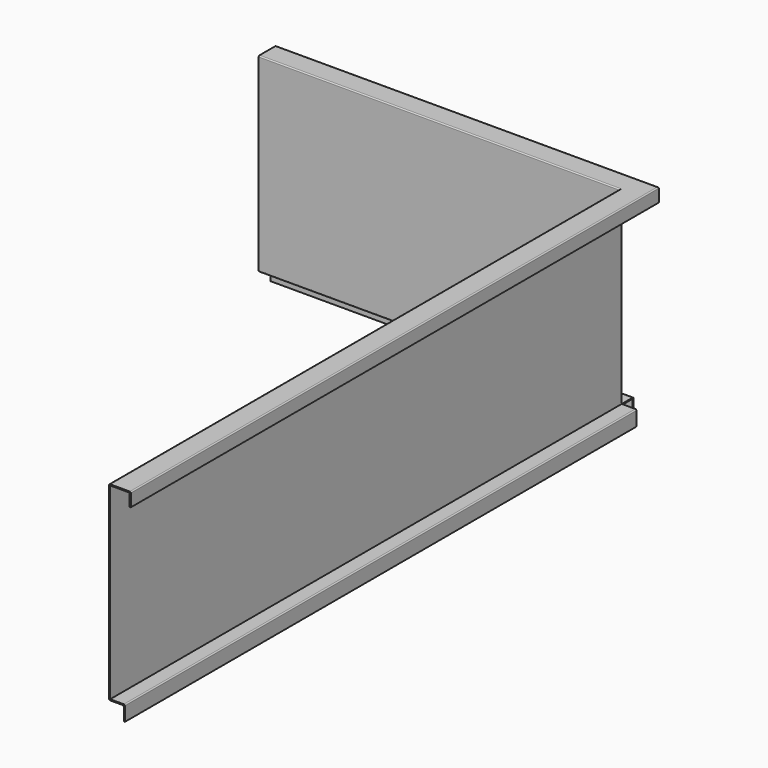
from build123d import *

# Parameters (mm, degrees)
F3_W         = 27
F3_H         = 27
F4_DEPTH     = 30
F5_T1_DEPTH  = 666
F5_T3_DEPTH  = 702
F5_T5_DEPTH  = 1176
F5_T7_DEPTH  = 1212
F5_T13_DEPTH = 1181
F5_T17_DEPTH = 671
F5_T20_DEPTH = 669
F5_T22_DEPTH = 676
F5_T24_DEPTH = 714
F5_T26_DEPTH = 1224
F5_T28_DEPTH = 1179
F5_T30_DEPTH = 1186
F5_T36_DEPTH = 674
F5_T40_DEPTH = 1184
F5_T47_DEPTH = 674
F5_T51_DEPTH = 1184


# Not quite as in the source:
# - a fillet or chamfer that OpenCascade refuses, or shapes differently, is made with other operations: its cross-section is extruded or revolved along the edge and cut away or added


with BuildPart() as f2:
    # F2: sweep along a path in F1
    with BuildLine(Plane.XY) as f2_path:
        Line((0, 0), (0, 1174))
        Line((0, 1174), (-664, 1174))
    # F0 (on Front) → F2 (sweep)
    with BuildSketch(Plane.XZ):
        Polygon((38, -2), (38, -25), (40, -25), (40, 0), (0, 0), (0, -350), (27, -350), (27, -376), (29, -376), (29, -348), (2, -348), (2, -2), align=None)
    sweep(path=f2_path.line, transition=Transition.RIGHT)

    # F3 (on face) → F4 (cut)
    with BuildSketch(Plane.XY.offset(-348)):
        with Locations((15.5, 1189.5)):
            Rectangle(F3_W, F3_H)
    extrude(amount=-F4_DEPTH, mode=Mode.SUBTRACT)

    # F5: fillet of radius 2 on 15 edges, made by hand

    # F5_s2 → F5_t1 (join)
    with BuildSketch(Plane.YZ.offset(-664)):
        with BuildLine():
            ThreePointArc((1199, -350), (1200.4142135624, -350.5857864376), (1201, -352))
            Line((1201, -352), (1201, -350))
            Line((1201, -350), (1199, -350))
        make_face()
        with BuildLine():
            ThreePointArc((1176, -346), (1176.5857864376, -347.4142135624), (1178, -348))
            Line((1178, -348), (1176, -348))
            Line((1176, -348), (1176, -346))
        make_face()
        with BuildLine():
            ThreePointArc((1178, -2), (1176.5857864376, -2.5857864376), (1176, -4))
            Line((1176, -4), (1176, -2))
            Line((1176, -2), (1178, -2))
        make_face()
    extrude(amount=F5_T1_DEPTH)

    # F5_s4 → F5_t3 (join)
    with BuildSketch(Plane.YZ.offset(-664)):
        with BuildLine():
            ThreePointArc((1210, -2), (1211.4142135624, -2.5857864376), (1212, -4))
            Line((1212, -4), (1212, -2))
            Line((1212, -2), (1210, -2))
        make_face()
    extrude(amount=F5_T3_DEPTH)

    # F5_s6 → F5_t5 (join)
    with BuildSketch(Plane.XZ.offset(-1176)):
        with BuildLine():
            ThreePointArc((25, -350), (26.4142135624, -350.5857864376), (27, -352))
            Line((27, -352), (27, -350))
            Line((27, -350), (25, -350))
        make_face()
        with BuildLine():
            ThreePointArc((4, -2), (2.5857864376, -2.5857864376), (2, -4))
            Line((2, -4), (2, -2))
            Line((2, -2), (4, -2))
        make_face()
    extrude(amount=F5_T5_DEPTH)

    # F5_s8 → F5_t7 (join)
    with BuildSketch(Plane.XZ.offset(-1212)):
        with BuildLine():
            ThreePointArc((38, -4), (37.4142135624, -2.5857864376), (36, -2))
            Line((36, -2), (38, -2))
            Line((38, -2), (38, -4))
        make_face()
    extrude(amount=F5_T7_DEPTH)


with BuildPart() as f5_tool11:
    # F5_s12 → F5_t13 (new body)
    with BuildSketch(Plane.XZ):
        with BuildLine():
            ThreePointArc((4, -2), (2.5857864376, -2.5857864376), (2, -4))
            Line((2, -4), (2, -2))
            Line((2, -2), (4, -2))
        make_face()
    extrude(amount=-F5_T13_DEPTH)

    split(bisect_by=Plane.XZ.offset(-1176), keep=Keep.BOTTOM)


with BuildPart() as f5_tool15:
    # F5_s16 → F5_t17 (new body)
    with BuildSketch(Plane.YZ.offset(7)):
        with BuildLine():
            ThreePointArc((1178, -2), (1176.5857864376, -2.5857864376), (1176, -4))
            Line((1176, -4), (1176, -2))
            Line((1176, -2), (1178, -2))
        make_face()
    extrude(amount=-F5_T17_DEPTH)

    split(bisect_by=Plane.YZ.offset(2), keep=Keep.TOP)


with BuildPart() as f5_tool11_1:
    add(f5_tool11.part)

    # F5_t19: intersect F5_tool15
    add(f5_tool15.part, mode=Mode.INTERSECT)


with BuildPart() as f2_1:
    add(f2.part)

    # F5_t9: union F5_tool11
    add(f5_tool11_1.part)

    # F5_s21 → F5_t20 (cut)
    with BuildSketch(Plane.YZ.offset(-669)):
        with BuildLine():
            ThreePointArc((1174, -348), (1174.5857864376, -349.4142135624), (1176, -350))
            Line((1176, -350), (1174, -350))
            Line((1174, -350), (1174, -348))
        make_face()
        with BuildLine():
            ThreePointArc((1174, -2), (1174.5857864376, -0.5857864376), (1176, 0))
            Line((1176, 0), (1174, 0))
            Line((1174, 0), (1174, -2))
        make_face()
    extrude(amount=F5_T20_DEPTH, mode=Mode.SUBTRACT)

    # F5_s23 → F5_t22 (cut)
    with BuildSketch(Plane.YZ.offset(-669)):
        with BuildLine():
            ThreePointArc((1201, -348), (1202.4142135624, -348.5857864376), (1203, -350))
            Line((1203, -350), (1203, -348))
            Line((1203, -348), (1201, -348))
        make_face()
    extrude(amount=F5_T22_DEPTH, mode=Mode.SUBTRACT)

    # F5_s25 → F5_t24 (cut)
    with BuildSketch(Plane.YZ.offset(-669)):
        with BuildLine():
            ThreePointArc((1214, -2), (1213.4142135624, -0.5857864376), (1212, 0))
            Line((1212, 0), (1214, 0))
            Line((1214, 0), (1214, -2))
        make_face()
    extrude(amount=F5_T24_DEPTH, mode=Mode.SUBTRACT)

    # F5_s27 → F5_t26 (cut)
    with BuildSketch(Plane.XZ.offset(-1219)):
        with BuildLine():
            ThreePointArc((38, 0), (39.4142135624, -0.5857864376), (40, -2))
            Line((40, -2), (40, 0))
            Line((40, 0), (38, 0))
        make_face()
    extrude(amount=F5_T26_DEPTH, mode=Mode.SUBTRACT)

    # F5_s29 → F5_t28 (cut)
    with BuildSketch(Plane.XZ.offset(-1174)):
        with BuildLine():
            ThreePointArc((0, -2), (0.5857864376, -0.5857864376), (2, 0))
            Line((2, 0), (0, 0))
            Line((0, 0), (0, -2))
        make_face()
        with BuildLine():
            ThreePointArc((2, -350), (0.5857864376, -349.4142135624), (0, -348))
            Line((0, -348), (0, -350))
            Line((0, -350), (2, -350))
        make_face()
    extrude(amount=F5_T28_DEPTH, mode=Mode.SUBTRACT)

    # F5_s31 → F5_t30 (cut)
    with BuildSketch(Plane.XZ.offset(-1181)):
        with BuildLine():
            ThreePointArc((27, -348), (28.4142135624, -348.5857864376), (29, -350))
            Line((29, -350), (29, -348))
            Line((29, -348), (27, -348))
        make_face()
    extrude(amount=F5_T30_DEPTH, mode=Mode.SUBTRACT)


with BuildPart() as f5_tool34:
    # F5_s35 → F5_t36 (new body)
    with BuildSketch(Plane.YZ.offset(5)):
        with BuildLine():
            ThreePointArc((1174, -348), (1174.5857864376, -349.4142135624), (1176, -350))
            Line((1176, -350), (1174, -350))
            Line((1174, -350), (1174, -348))
        make_face()
    extrude(amount=-F5_T36_DEPTH)

    split(bisect_by=Plane.YZ, keep=Keep.TOP)


with BuildPart() as f5_tool38:
    # F5_s39 → F5_t40 (new body)
    with BuildSketch(Plane.XZ.offset(5)):
        with BuildLine():
            ThreePointArc((2, -350), (0.5857864376, -349.4142135624), (0, -348))
            Line((0, -348), (0, -350))
            Line((0, -350), (2, -350))
        make_face()
    extrude(amount=-F5_T40_DEPTH)

    split(bisect_by=Plane.XZ.offset(-1174), keep=Keep.BOTTOM)


with BuildPart() as f5_tool34_1:
    add(f5_tool34.part)

    # F5_t42: intersect F5_tool38
    add(f5_tool38.part, mode=Mode.INTERSECT)


with BuildPart() as f2_2:
    add(f2_1.part)

    # F5_t32: cut F5_tool34
    add(f5_tool34_1.part, mode=Mode.SUBTRACT)


with BuildPart() as f5_tool45:
    # F5_s46 → F5_t47 (new body)
    with BuildSketch(Plane.YZ.offset(5)):
        with BuildLine():
            ThreePointArc((1174, -2), (1174.5857864376, -0.5857864376), (1176, 0))
            Line((1176, 0), (1174, 0))
            Line((1174, 0), (1174, -2))
        make_face()
    extrude(amount=-F5_T47_DEPTH)

    split(bisect_by=Plane.YZ, keep=Keep.TOP)


with BuildPart() as f5_tool49:
    # F5_s50 → F5_t51 (new body)
    with BuildSketch(Plane.XZ.offset(5)):
        with BuildLine():
            ThreePointArc((0, -2), (0.5857864376, -0.5857864376), (2, 0))
            Line((2, 0), (0, 0))
            Line((0, 0), (0, -2))
        make_face()
    extrude(amount=-F5_T51_DEPTH)

    split(bisect_by=Plane.XZ.offset(-1174), keep=Keep.BOTTOM)


with BuildPart() as f5_tool45_1:
    add(f5_tool45.part)

    # F5_t53: intersect F5_tool49
    add(f5_tool49.part, mode=Mode.INTERSECT)


with BuildPart() as f2_3:
    add(f2_2.part)

    # F5_t43: cut F5_tool45
    add(f5_tool45_1.part, mode=Mode.SUBTRACT)


solid = f2_3.part
